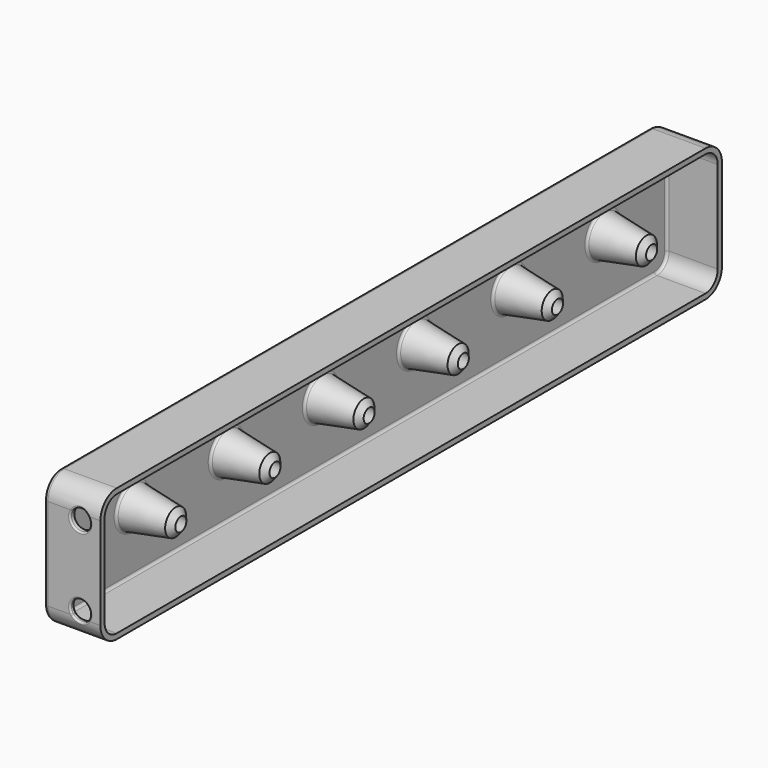
from build123d import *

# Parameters (mm, degrees)
F0_W         = 915
F0_H         = 165.1
F1_DEPTH     = 70
F2_DEPTH     = 36.63
F3_DEPTH     = 12.5
F4_R         = 20.32
F5_DEPTH     = 70.001
F5_TAPER     = 10
F6_R         = 5
F7_T1_DEPTH  = 133.5
F7_T4_ANGLE  = 90
F7_T6_ANGLE  = 90
F7_T8_ANGLE  = 90
F7_T10_ANGLE = 90
F8_T         = -6.5
F9_R         = 3.175
F12_DEPTH    = 25
F13_R        = 2


# Not quite as in the source:
# - a fillet or chamfer that OpenCascade refuses, or shapes differently, is made with other operations: its cross-section is extruded or revolved along the edge and cut away or added


with BuildPart() as f1:
    # F0 (on Right) → F1 (new body)
    with BuildSketch(Plane.YZ):
        Rectangle(F0_W, F0_H)
    extrude(amount=F1_DEPTH)

    # F2 (add): a face of the model
    f2_faces = [f1.faces().sort_by_distance(p)[0] for p in [
        (35, -457.5, 0),
    ]]
    extrude(f2_faces, amount=F2_DEPTH)

    # F3 (add): a face of the model
    f3_faces = [f1.faces().sort_by_distance(p)[0] for p in [
        (35, 457.5, 0),
    ]]
    extrude(f3_faces, amount=F3_DEPTH)

    # F4 (on face) → F5 (cut, through all)
    with BuildSketch(Plane.YZ):
        with Locations((-365.125, 0)):
            Circle(F4_R)
        with Locations((-73.025, 0)):
            Circle(F4_R)
        with Locations((73.025, 0)):
            Circle(F4_R)
        with Locations((-219.075, 0)):
            Circle(F4_R)
        with Locations((219.075, 0)):
            Circle(F4_R)
        with Locations((365.125, 0)):
            Circle(F4_R)
    extrude(amount=F5_DEPTH, taper=F5_TAPER, mode=Mode.SUBTRACT)

    # F6
    f6_edges = [f1.edges().sort_by_distance(p)[0] for p in [
        (0, -494.13, 0),
        (0, -12.065, 82.55),
        (0, -12.065, -82.55),
        (0, 470, 0),
        (0, -385.445, 0),
        (0, -239.395, 0),
        (0, -93.345, 0),
        (0, 52.705, 0),
        (0, 198.755, 0),
        (0, 344.805, 0),
    ]]
    fillet(f6_edges, radius=F6_R)

    # F7: fillet of radius 25.4 on 4 edges, made by hand

    # F7_s2 → F7_t1 (cut)
    with BuildSketch(Plane.YZ):
        with BuildLine():
            ThreePointArc((-468.73, 82.55), (-486.6905122421, 75.1105122421), (-494.13, 57.15))
            Line((-494.13, 57.15), (-494.13, 82.55))
            Line((-494.13, 82.55), (-468.73, 82.55))
        make_face()
        with BuildLine():
            ThreePointArc((-494.13, -57.15), (-486.6905122421, -75.1105122421), (-468.73, -82.55))
            Line((-468.73, -82.55), (-494.13, -82.55))
            Line((-494.13, -82.55), (-494.13, -57.15))
        make_face()
        with BuildLine():
            ThreePointArc((470, -57.15), (462.5605122421, -75.1105122421), (444.6, -82.55))
            Line((444.6, -82.55), (470, -82.55))
            Line((470, -82.55), (470, -57.15))
        make_face()
        with BuildLine():
            ThreePointArc((444.6, 82.55), (462.5605122421, 75.1105122421), (470, 57.15))
            Line((470, 57.15), (470, 82.55))
            Line((470, 82.55), (444.6, 82.55))
        make_face()
    extrude(amount=F7_T1_DEPTH, mode=Mode.SUBTRACT)

    # F7_s3 → F7_t4 (revolve, cut)
    with BuildSketch(Plane.XZ.offset(-444.6)):
        with BuildLine():
            ThreePointArc((0, 77.55), (1.4644660941, 81.0855339059), (5, 82.55))
            Line((5, 82.55), (0, 82.55))
            Line((0, 82.55), (0, 77.55))
        make_face()
    revolve(axis=Axis((0, 444.6, 57.15), (-1, 0, 0)), revolution_arc=F7_T4_ANGLE, mode=Mode.SUBTRACT)

    # F7_s5 → F7_t6 (revolve, cut)
    with BuildSketch(Plane.XY.offset(-57.15)):
        with BuildLine():
            ThreePointArc((0, 465), (1.4644660941, 468.5355339059), (5, 470))
            Line((5, 470), (0, 470))
            Line((0, 470), (0, 465))
        make_face()
    revolve(axis=Axis((0, 444.6, -57.15), (-1, 0, 0)), revolution_arc=F7_T6_ANGLE, mode=Mode.SUBTRACT)

    # F7_s7 → F7_t8 (revolve, cut)
    with BuildSketch(Plane.XZ.offset(468.73)):
        with BuildLine():
            ThreePointArc((0, -77.55), (1.4644660941, -81.0855339059), (5, -82.55))
            Line((5, -82.55), (0, -82.55))
            Line((0, -82.55), (0, -77.55))
        make_face()
    revolve(axis=Axis((0, -468.73, -57.15), (-1, 0, 0)), revolution_arc=F7_T8_ANGLE, mode=Mode.SUBTRACT)

    # F7_s9 → F7_t10 (revolve, cut)
    with BuildSketch(Plane.XY.offset(57.15)):
        with BuildLine():
            ThreePointArc((0, -489.13), (1.4644660941, -492.6655339059), (5, -494.13))
            Line((5, -494.13), (0, -494.13))
            Line((0, -494.13), (0, -489.13))
        make_face()
    revolve(axis=Axis((0, -468.73, 57.15), (-1, 0, 0)), revolution_arc=F7_T10_ANGLE, mode=Mode.SUBTRACT)

    # F8
    f8_openings = [f1.faces().sort_by_distance(p)[0] for p in [
        (70, -12.156928, 0),
    ]]
    offset(amount=F8_T, openings=f8_openings, kind=Kind.INTERSECTION)

    # F9
    f9_edges = [f1.edges().sort_by_distance(p)[0] for p in [
        (6.5, 339.350852, 0),
        (6.5, -390.899148, 0),
        (6.5, -12.065, -76.05),
        (6.5, 457.964318, -70.514318),
        (6.5, 463.5, 0),
        (6.5, 457.964318, 70.514318),
        (6.5, -12.065, 76.05),
        (6.5, -482.094318, 70.514318),
        (6.5, -487.63, 0),
        (6.5, -482.094318, -70.514318),
        (6.5, 193.300852, 0),
        (6.5, 47.250852, 0),
        (6.5, -98.799148, 0),
        (6.5, -244.849148, 0),
    ]]
    fillet(f9_edges, radius=F9_R)

    # F10: chamfer of 10 on 6 edges, made by hand

    # F10_s1 → F10_t2 (revolve, cut)
    with BuildSketch(Plane.XY):
        Polygon((60.1519224699, 381.4388661043), (70, 369.7023843277), (70, 379.7023843277), align=None)
    revolve(axis=Axis((70, 365.125, 0), (1, 0, 0)), mode=Mode.SUBTRACT)

    # F10_s3 → F10_t4 (revolve, cut)
    with BuildSketch(Plane.XY):
        Polygon((60.1519224699, -348.8111338957), (70, -360.5476156723), (70, -350.5476156723), align=None)
    revolve(axis=Axis((70, -365.125, 0), (1, 0, 0)), mode=Mode.SUBTRACT)

    # F10_s5 → F10_t6 (revolve, cut)
    with BuildSketch(Plane.XY):
        Polygon((60.1519224699, 235.3888661043), (70, 223.6523843277), (70, 233.6523843277), align=None)
    revolve(axis=Axis((70, 219.075, 0), (1, 0, 0)), mode=Mode.SUBTRACT)

    # F10_s7 → F10_t8 (revolve, cut)
    with BuildSketch(Plane.XY):
        Polygon((60.1519224699, 89.3388661043), (70, 77.6023843277), (70, 87.6023843277), align=None)
    revolve(axis=Axis((70, 73.025, 0), (1, 0, 0)), mode=Mode.SUBTRACT)

    # F10_s9 → F10_t10 (revolve, cut)
    with BuildSketch(Plane.XY):
        Polygon((60.1519224699, -56.7111338957), (70, -68.4476156723), (70, -58.4476156723), align=None)
    revolve(axis=Axis((70, -73.025, 0), (1, 0, 0)), mode=Mode.SUBTRACT)

    # F10_s11 → F10_t12 (revolve, cut)
    with BuildSketch(Plane.XY):
        Polygon((60.1519224699, -202.7611338957), (70, -214.4976156723), (70, -204.4976156723), align=None)
    revolve(axis=Axis((70, -219.075, 0), (1, 0, 0)), mode=Mode.SUBTRACT)

    # F11 (on face) → F12 (cut)
    with BuildSketch(Plane.XZ.offset(494.13)):
        with BuildLine():
            Line((54.807522623, -57.15), (35.192477377, -57.15))
            ThreePointArc((35.192477377, -57.15), (45, -61.9), (54.807522623, -57.15))
        make_face()
        with BuildLine():
            ThreePointArc((54.807522623, -57.15), (56.8077100402, -53.5021925365), (57.5, -49.4))
            ThreePointArc((57.5, -49.4), (40.8978074635, -37.5922899598), (35.192477377, -57.15))
            Line((35.192477377, -57.15), (54.807522623, -57.15))
        make_face()
        with BuildLine():
            Line((54.807522623, 57.15), (35.192477377, 57.15))
            ThreePointArc((35.192477377, 57.15), (40.8978074635, 37.5922899598), (57.5, 49.4))
            ThreePointArc((57.5, 49.4), (56.8077100402, 53.5021925365), (54.807522623, 57.15))
        make_face()
        with BuildLine():
            ThreePointArc((54.807522623, 57.15), (45, 61.9), (35.192477377, 57.15))
            Line((35.192477377, 57.15), (54.807522623, 57.15))
        make_face()
    extrude(amount=-F12_DEPTH, mode=Mode.SUBTRACT)

    # F13
    f13_edges = [f1.edges().sort_by_distance(p)[0] for p in [
        (45, -487.63, -36.9),
        (45, -494.13, 36.9),
        (45, -493.681904, -61.9),
        (45, -493.681904, 61.9),
        (44.999944, -487.023373, -61.9),
        (45, -494.13, -36.9),
    ]]
    fillet(f13_edges, radius=F13_R)


solid = f1.part
